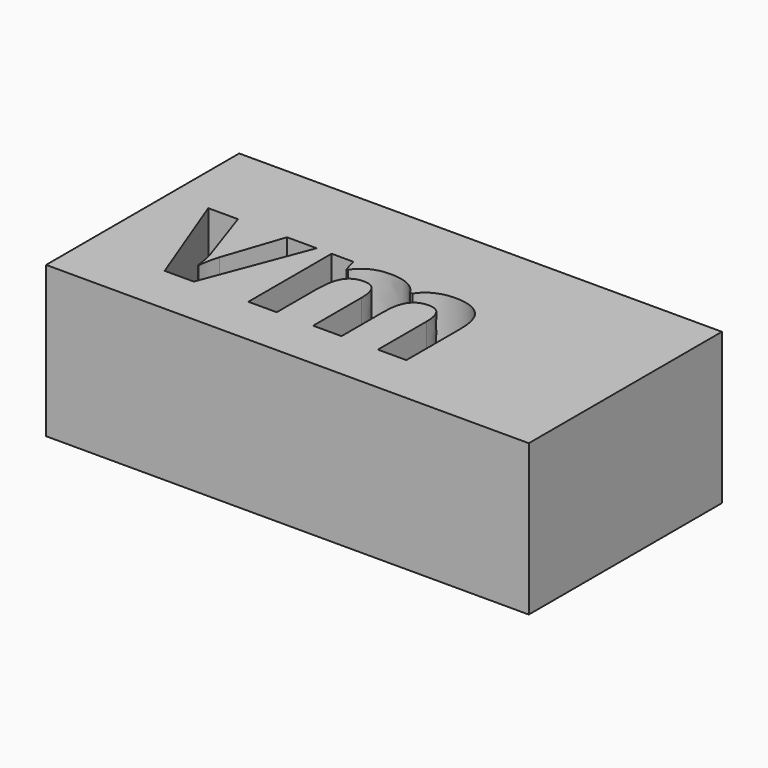
from build123d import *

# Parameters (mm, degrees)
F0_W         = 80
F0_H         = 40
F1_DEPTH     = 25
F2_TEXT_SIZE = 31.5842257502
F3_DEPTH     = 35


# Not quite as in the source:
# - Text() gives the source's letters only with a copy of the font that has no kerning and outlines rounded to 1/6400 em; it was checked with that copy


with BuildPart() as f1:
    # F0 (on Top) → F1 (new body)
    with BuildSketch(Plane.XY):
        with Locations((40, 20)):
            Rectangle(F0_W, F0_H)
    extrude(amount=-F1_DEPTH)

    # F2 (on face) → F3 (cut)
    with BuildSketch(Plane.XY):
        with Locations((6.457219366, 8.2820849493)):
            Text('vm', F2_TEXT_SIZE, font='Open Sans', font_style=FontStyle.BOLD, text_align=(TextAlign.LEFT, TextAlign.BOTTOM))
    extrude(amount=-F3_DEPTH, mode=Mode.SUBTRACT)


solid = f1.part
